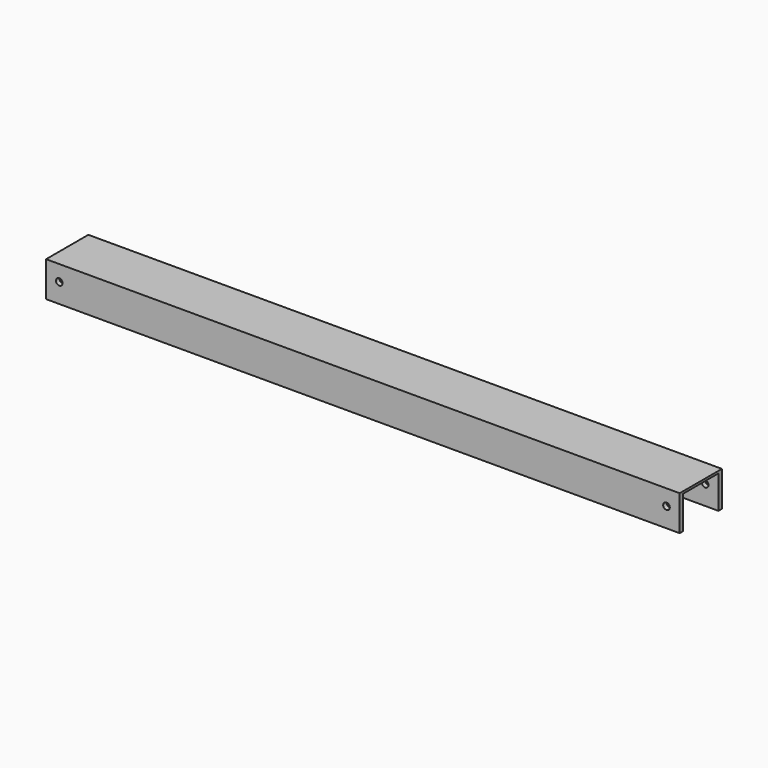
from build123d import *

# Parameters (mm, degrees)
F0_W     = 914.4
F0_H     = 50.8
F1_DEPTH = 6.35
F2_W     = 914.4
F2_H     = 69.85
F3_DEPTH = 3.175
F4_W     = 914.4
F4_H     = 6.35
F5_DEPTH = 47.625
F7_D     = 9.525


with BuildPart() as f1:
    # F0 (on Front) → F1 (new body)
    with BuildSketch(Plane.XZ):
        with Locations((564.6889274399, 584.2)):
            Rectangle(F0_W, F0_H)
    extrude(amount=F1_DEPTH)

    # F2 (on face) → F3 (join)
    with BuildSketch(Plane.XY.offset(609.6)):
        with Locations((564.6889274399, 34.925)):
            Rectangle(F2_W, F2_H)
    extrude(amount=-F3_DEPTH)

    # F4 (on face) → F5 (join, through all)
    with BuildSketch(Plane(origin=(0, 0, 606.425), x_dir=(1, 0, 0), z_dir=(0, 0, -1))):
        with Locations((564.6889274399, -66.675)):
            Rectangle(F4_W, F4_H)
    extrude(amount=F5_DEPTH)

    # F7 (through all)
    with Locations(Plane.XZ.offset(6.35)):
        with Locations((126.5389274399, 586.8924), (1002.8389274399, 586.8924)):
            Hole(F7_D / 2)


solid = f1.part
